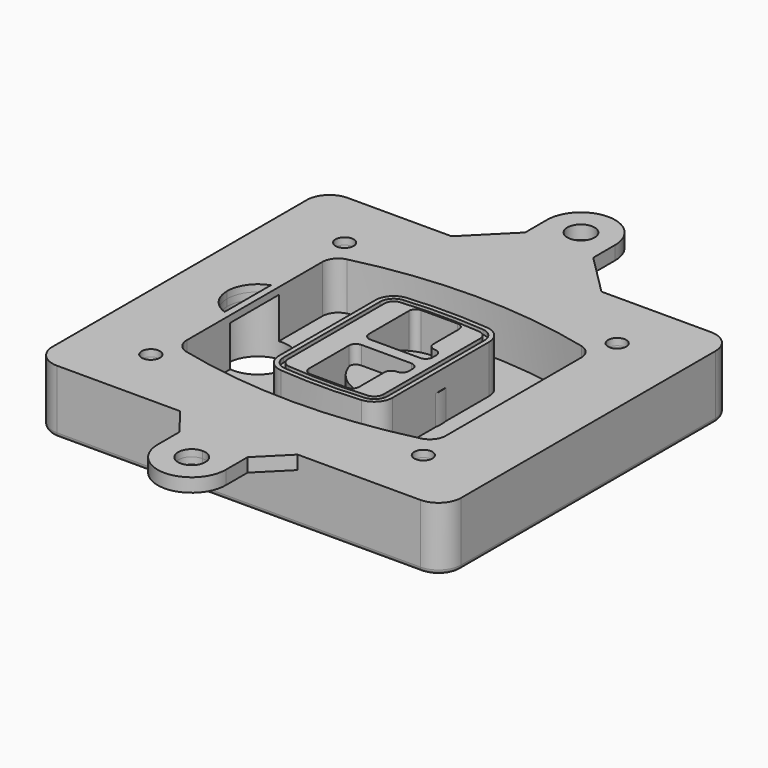
from build123d import *

# Parameters (mm, degrees)
F0_R      = 4
F1_DEPTH  = 25
F2_DEPTH  = 3
F3_DEPTH  = 18
F5_DEPTH  = 21
F6_DEPTH  = 2
F8_DEPTH  = 20
F9_DEPTH  = 16
F10_DEPTH = 25
F7_R      = 6
F7_R_2    = 4
F11_DEPTH = 6
F13_DEPTH = 9
F15_R     = 2
F16_R     = 4
F17_DEPTH = 3


# Not quite as in the source:
# - a feature of the source that left no trace in its solid (it failed there, or was rolled back) is left out
# - a feature names something its author has since deleted; it is built from what else it names


with BuildPart() as f1:
    # F0 (on Top) → F1 (new body)
    with BuildSketch(Plane.XY):
        with BuildLine():
            ThreePointArc((-90, -70), (-87.0710678119, -77.0710678119), (-80, -80))
            Line((-80, -80), (80, -80))
            ThreePointArc((80, -80), (87.0710678119, -77.0710678119), (90, -70))
            Line((90, -70), (90, 70))
            ThreePointArc((90, 70), (87.0710678119, 77.0710678119), (80, 80))
            Line((80, 80), (-80, 80))
            ThreePointArc((-80, 80), (-87.0710678119, 77.0710678119), (-90, 70))
            Line((-90, 70), (-90, -70))
        make_face()
        with Locations((-60, -53.3333333333)):
            Circle(F0_R, mode=Mode.SUBTRACT)
        with Locations((60, -53.3333333333)):
            Circle(F0_R, mode=Mode.SUBTRACT)
        with Locations((-60, 53.3333333333)):
            Circle(F0_R, mode=Mode.SUBTRACT)
        with BuildLine():
            ThreePointArc((-64, 37.2990447398), (-61.0143011354, 45.9411029726), (-53.3306899286, 50.8970778549))
            ThreePointArc((-53.3306899286, 50.8970778549), (0, 57.3333333333), (53.3306899286, 50.8970778549))
            ThreePointArc((53.3306899286, 50.8970778549), (61.0143011354, 45.9411029726), (64, 37.2990447398))
            Line((64, 37.2990447398), (64, -37.2990447398))
            ThreePointArc((64, -37.2990447398), (61.0143011354, -45.9411029726), (53.3306899286, -50.8970778549))
            ThreePointArc((53.3306899286, -50.8970778549), (0, -57.3333333333), (-53.3306899286, -50.8970778549))
            ThreePointArc((-53.3306899286, -50.8970778549), (-61.0143011354, -45.9411029726), (-64, -37.2990447398))
            Line((-64, -37.2990447398), (-64, 37.2990447398))
        make_face(mode=Mode.SUBTRACT)
        with Locations((60, 53.3333333333)):
            Circle(F0_R, mode=Mode.SUBTRACT)
        with BuildLine():
            ThreePointArc((53.3306899286, 50.8970778549), (0, 57.3333333333), (-53.3306899286, 50.8970778549))
            ThreePointArc((-53.3306899286, 50.8970778549), (-61.0143011354, 45.9411029726), (-64, 37.2990447398))
            Line((-64, 37.2990447398), (-64, -37.2990447398))
            ThreePointArc((-64, -37.2990447398), (-61.0143011354, -45.9411029726), (-53.3306899286, -50.8970778549))
            ThreePointArc((-53.3306899286, -50.8970778549), (0, -57.3333333333), (53.3306899286, -50.8970778549))
            ThreePointArc((53.3306899286, -50.8970778549), (61.0143011354, -45.9411029726), (64, -37.2990447398))
            Line((64, -37.2990447398), (64, 37.2990447398))
            ThreePointArc((64, 37.2990447398), (61.0143011354, 45.9411029726), (53.3306899286, 50.8970778549))
        make_face()
        with BuildLine():
            Line((-60, -37.2990447398), (-60, 37.2990447398))
            ThreePointArc((-60, 37.2990447398), (-57.8673579538, 43.4719434775), (-52.3790642347, 47.0119255363))
            ThreePointArc((-52.3790642347, 47.0119255363), (0, 53.3333333333), (52.3790642347, 47.0119255363))
            ThreePointArc((52.3790642347, 47.0119255363), (57.8673579538, 43.4719434775), (60, 37.2990447398))
            Line((60, 37.2990447398), (60, -37.2990447398))
            ThreePointArc((60, -37.2990447398), (57.8673579538, -43.4719434775), (52.3790642347, -47.0119255363))
            ThreePointArc((52.3790642347, -47.0119255363), (0, -53.3333333333), (-52.3790642347, -47.0119255363))
            ThreePointArc((-52.3790642347, -47.0119255363), (-57.8673579538, -43.4719434775), (-60, -37.2990447398))
        make_face(mode=Mode.SUBTRACT)
        with BuildLine():
            ThreePointArc((-52.3790642347, 47.0119255363), (-57.8673579538, 43.4719434775), (-60, 37.2990447398))
            Line((-60, 37.2990447398), (-60, -37.2990447398))
            ThreePointArc((-60, -37.2990447398), (-57.8673579538, -43.4719434775), (-52.3790642347, -47.0119255363))
            ThreePointArc((-52.3790642347, -47.0119255363), (0, -53.3333333333), (52.3790642347, -47.0119255363))
            ThreePointArc((52.3790642347, -47.0119255363), (57.8673579538, -43.4719434775), (60, -37.2990447398))
            Line((60, -37.2990447398), (60, 37.2990447398))
            ThreePointArc((60, 37.2990447398), (57.8673579538, 43.4719434775), (52.3790642347, 47.0119255363))
            ThreePointArc((52.3790642347, 47.0119255363), (0, 53.3333333333), (-52.3790642347, 47.0119255363))
        make_face()
        with BuildLine():
            ThreePointArc((51.6653449643, 44.0980612973), (55.5071505677, 41.6200738562), (57, 37.2990447398))
            Line((57, 37.2990447398), (57, -37.2990447398))
            ThreePointArc((57, -37.2990447398), (55.5071505677, -41.6200738562), (51.6653449643, -44.0980612973))
            ThreePointArc((51.6653449643, -44.0980612973), (0, -50.3333333333), (-51.6653449643, -44.0980612973))
            ThreePointArc((-51.6653449643, -44.0980612973), (-55.5071505677, -41.6200738562), (-57, -37.2990447398))
            Line((-57, -37.2990447398), (-57, 37.2990447398))
            ThreePointArc((-57, 37.2990447398), (-55.5071505677, 41.6200738562), (-51.6653449643, 44.0980612973))
            ThreePointArc((-51.6653449643, 44.0980612973), (0, 50.3333333333), (51.6653449643, 44.0980612973))
        make_face(mode=Mode.SUBTRACT)
        with BuildLine():
            Line((57, -37.2990447398), (57, 37.2990447398))
            ThreePointArc((57, 37.2990447398), (55.5071505677, 41.6200738562), (51.6653449643, 44.0980612973))
            ThreePointArc((51.6653449643, 44.0980612973), (0, 50.3333333333), (-51.6653449643, 44.0980612973))
            ThreePointArc((-51.6653449643, 44.0980612973), (-55.5071505677, 41.6200738562), (-57, 37.2990447398))
            Line((-57, 37.2990447398), (-57, -37.2990447398))
            ThreePointArc((-57, -37.2990447398), (-55.5071505677, -41.6200738562), (-51.6653449643, -44.0980612973))
            ThreePointArc((-51.6653449643, -44.0980612973), (0, -50.3333333333), (51.6653449643, -44.0980612973))
            ThreePointArc((51.6653449643, -44.0980612973), (55.5071505677, -41.6200738562), (57, -37.2990447398))
        make_face()
    extrude(amount=-F1_DEPTH)

    # F0 (on Top) → F2 (join)
    with BuildSketch(Plane.XY):
        with BuildLine():
            ThreePointArc((-52.3790642347, 47.0119255363), (-57.8673579538, 43.4719434775), (-60, 37.2990447398))
            Line((-60, 37.2990447398), (-60, -37.2990447398))
            ThreePointArc((-60, -37.2990447398), (-57.8673579538, -43.4719434775), (-52.3790642347, -47.0119255363))
            ThreePointArc((-52.3790642347, -47.0119255363), (0, -53.3333333333), (52.3790642347, -47.0119255363))
            ThreePointArc((52.3790642347, -47.0119255363), (57.8673579538, -43.4719434775), (60, -37.2990447398))
            Line((60, -37.2990447398), (60, 37.2990447398))
            ThreePointArc((60, 37.2990447398), (57.8673579538, 43.4719434775), (52.3790642347, 47.0119255363))
            ThreePointArc((52.3790642347, 47.0119255363), (0, 53.3333333333), (-52.3790642347, 47.0119255363))
        make_face()
        with BuildLine():
            ThreePointArc((51.6653449643, 44.0980612973), (55.5071505677, 41.6200738562), (57, 37.2990447398))
            Line((57, 37.2990447398), (57, -37.2990447398))
            ThreePointArc((57, -37.2990447398), (55.5071505677, -41.6200738562), (51.6653449643, -44.0980612973))
            ThreePointArc((51.6653449643, -44.0980612973), (0, -50.3333333333), (-51.6653449643, -44.0980612973))
            ThreePointArc((-51.6653449643, -44.0980612973), (-55.5071505677, -41.6200738562), (-57, -37.2990447398))
            Line((-57, -37.2990447398), (-57, 37.2990447398))
            ThreePointArc((-57, 37.2990447398), (-55.5071505677, 41.6200738562), (-51.6653449643, 44.0980612973))
            ThreePointArc((-51.6653449643, 44.0980612973), (0, 50.3333333333), (51.6653449643, 44.0980612973))
        make_face(mode=Mode.SUBTRACT)
    extrude(amount=F2_DEPTH)

    # F0 (on Top) → F3 (cut)
    with BuildSketch(Plane.XY):
        with BuildLine():
            Line((57, -37.2990447398), (57, 37.2990447398))
            ThreePointArc((57, 37.2990447398), (55.5071505677, 41.6200738562), (51.6653449643, 44.0980612973))
            ThreePointArc((51.6653449643, 44.0980612973), (0, 50.3333333333), (-51.6653449643, 44.0980612973))
            ThreePointArc((-51.6653449643, 44.0980612973), (-55.5071505677, 41.6200738562), (-57, 37.2990447398))
            Line((-57, 37.2990447398), (-57, -37.2990447398))
            ThreePointArc((-57, -37.2990447398), (-55.5071505677, -41.6200738562), (-51.6653449643, -44.0980612973))
            ThreePointArc((-51.6653449643, -44.0980612973), (0, -50.3333333333), (51.6653449643, -44.0980612973))
            ThreePointArc((51.6653449643, -44.0980612973), (55.5071505677, -41.6200738562), (57, -37.2990447398))
        make_face()
    extrude(amount=-F3_DEPTH, mode=Mode.SUBTRACT)

    # F4 (on face) → F5 (join, through all)
    with BuildSketch(Plane.XY.offset(3)):
        with BuildLine():
            ThreePointArc((-25, -26.587695628), (-22.8992979869, -31.9912392117), (-17.7004291845, -34.5569740744))
            ThreePointArc((-17.7004291845, -34.5569740744), (0, -35.3333333333), (17.7004291845, -34.5569740744))
            ThreePointArc((17.7004291845, -34.5569740744), (22.8992979869, -31.9912392117), (25, -26.587695628))
            Line((25, -26.587695628), (25, 26.587695628))
            ThreePointArc((25, 26.587695628), (22.8992979869, 31.9912392117), (17.7004291845, 34.5569740744))
            ThreePointArc((17.7004291845, 34.5569740744), (0, 35.3333333333), (-17.7004291845, 34.5569740744))
            ThreePointArc((-17.7004291845, 34.5569740744), (-22.8992979869, 31.9912392117), (-25, 26.587695628))
            Line((-25, 26.587695628), (-25, -26.587695628))
        make_face()
        with BuildLine():
            ThreePointArc((17.5253218884, 32.5646544628), (21.4244734902, 30.6403533158), (23, 26.587695628))
            Line((23, 26.587695628), (23, -26.587695628))
            ThreePointArc((23, -26.587695628), (21.4244734902, -30.6403533158), (17.5253218884, -32.5646544628))
            ThreePointArc((17.5253218884, -32.5646544628), (0, -33.3333333333), (-17.5253218884, -32.5646544628))
            ThreePointArc((-17.5253218884, -32.5646544628), (-21.4244734902, -30.6403533158), (-23, -26.587695628))
            Line((-23, -26.587695628), (-23, 26.587695628))
            ThreePointArc((-23, 26.587695628), (-21.4244734902, 30.6403533158), (-17.5253218884, 32.5646544628))
            ThreePointArc((-17.5253218884, 32.5646544628), (0, 33.3333333333), (17.5253218884, 32.5646544628))
        make_face(mode=Mode.SUBTRACT)
        with BuildLine():
            Line((23, -26.587695628), (23, 26.587695628))
            ThreePointArc((23, 26.587695628), (21.4244734902, 30.6403533158), (17.5253218884, 32.5646544628))
            ThreePointArc((17.5253218884, 32.5646544628), (0, 33.3333333333), (-17.5253218884, 32.5646544628))
            ThreePointArc((-17.5253218884, 32.5646544628), (-21.4244734902, 30.6403533158), (-23, 26.587695628))
            Line((-23, 26.587695628), (-23, -26.587695628))
            ThreePointArc((-23, -26.587695628), (-21.4244734902, -30.6403533158), (-17.5253218884, -32.5646544628))
            ThreePointArc((-17.5253218884, -32.5646544628), (0, -33.3333333333), (17.5253218884, -32.5646544628))
            ThreePointArc((17.5253218884, -32.5646544628), (21.4244734902, -30.6403533158), (23, -26.587695628))
        make_face()
        with BuildLine():
            ThreePointArc((17.3502145923, 30.5723348512), (19.9496489934, 29.2894674198), (21, 26.587695628))
            Line((21, 26.587695628), (21, -26.587695628))
            ThreePointArc((21, -26.587695628), (19.9496489934, -29.2894674198), (17.3502145923, -30.5723348512))
            ThreePointArc((17.3502145923, -30.5723348512), (0, -31.3333333333), (-17.3502145923, -30.5723348512))
            ThreePointArc((-17.3502145923, -30.5723348512), (-19.9496489934, -29.2894674198), (-21, -26.587695628))
            Line((-21, -26.587695628), (-21, 26.587695628))
            ThreePointArc((-21, 26.587695628), (-19.9496489934, 29.2894674198), (-17.3502145923, 30.5723348512))
            ThreePointArc((-17.3502145923, 30.5723348512), (0, 31.3333333333), (17.3502145923, 30.5723348512))
        make_face(mode=Mode.SUBTRACT)
        with BuildLine():
            Line((21, -26.587695628), (21, 26.587695628))
            ThreePointArc((21, 26.587695628), (19.9496489934, 29.2894674198), (17.3502145923, 30.5723348512))
            ThreePointArc((17.3502145923, 30.5723348512), (0, 31.3333333333), (-17.3502145923, 30.5723348512))
            ThreePointArc((-17.3502145923, 30.5723348512), (-19.9496489934, 29.2894674198), (-21, 26.587695628))
            Line((-21, 26.587695628), (-21, -26.587695628))
            ThreePointArc((-21, -26.587695628), (-19.9496489934, -29.2894674198), (-17.3502145923, -30.5723348512))
            ThreePointArc((-17.3502145923, -30.5723348512), (0, -31.3333333333), (17.3502145923, -30.5723348512))
            ThreePointArc((17.3502145923, -30.5723348512), (19.9496489934, -29.2894674198), (21, -26.587695628))
        make_face()
        with BuildLine():
            Line((-8, -2.5), (14, -2.5))
            ThreePointArc((14, -2.5), (16.1213203436, -3.3786796564), (17, -5.5))
            Line((17, -5.5), (17, -7.5))
            ThreePointArc((17, -7.5), (16.1213203436, -9.6213203436), (14, -10.5))
            ThreePointArc((14, -10.5), (11.8786796564, -11.3786796564), (11, -13.5))
            Line((11, -13.5), (11, -27.5))
            ThreePointArc((11, -27.5), (10.1213203436, -29.6213203436), (8, -30.5))
            Line((8, -30.5), (-8, -30.5))
            ThreePointArc((-8, -30.5), (-10.1213203436, -29.6213203436), (-11, -27.5))
            Line((-11, -27.5), (-11, -5.5))
            ThreePointArc((-11, -5.5), (-10.1213203436, -3.3786796564), (-8, -2.5))
        make_face(mode=Mode.SUBTRACT)
        with BuildLine():
            ThreePointArc((-8, 2.5), (-10.1213203436, 3.3786796564), (-11, 5.5))
            Line((-11, 5.5), (-11, 27.5))
            ThreePointArc((-11, 27.5), (-10.1213203436, 29.6213203436), (-8, 30.5))
            Line((-8, 30.5), (8, 30.5))
            ThreePointArc((8, 30.5), (10.1213203436, 29.6213203436), (11, 27.5))
            Line((11, 27.5), (11, 13.5))
            ThreePointArc((11, 13.5), (11.8786796564, 11.3786796564), (14, 10.5))
            ThreePointArc((14, 10.5), (16.1213203436, 9.6213203436), (17, 7.5))
            Line((17, 7.5), (17, 5.5))
            ThreePointArc((17, 5.5), (16.1213203436, 3.3786796564), (14, 2.5))
            Line((14, 2.5), (-8, 2.5))
        make_face(mode=Mode.SUBTRACT)
    extrude(amount=-F5_DEPTH)

    # F4 (on face) → F6 (cut)
    with BuildSketch(Plane.XY.offset(3)):
        with BuildLine():
            Line((23, -26.587695628), (23, 26.587695628))
            ThreePointArc((23, 26.587695628), (21.4244734902, 30.6403533158), (17.5253218884, 32.5646544628))
            ThreePointArc((17.5253218884, 32.5646544628), (0, 33.3333333333), (-17.5253218884, 32.5646544628))
            ThreePointArc((-17.5253218884, 32.5646544628), (-21.4244734902, 30.6403533158), (-23, 26.587695628))
            Line((-23, 26.587695628), (-23, -26.587695628))
            ThreePointArc((-23, -26.587695628), (-21.4244734902, -30.6403533158), (-17.5253218884, -32.5646544628))
            ThreePointArc((-17.5253218884, -32.5646544628), (0, -33.3333333333), (17.5253218884, -32.5646544628))
            ThreePointArc((17.5253218884, -32.5646544628), (21.4244734902, -30.6403533158), (23, -26.587695628))
        make_face()
        with BuildLine():
            ThreePointArc((17.3502145923, 30.5723348512), (19.9496489934, 29.2894674198), (21, 26.587695628))
            Line((21, 26.587695628), (21, -26.587695628))
            ThreePointArc((21, -26.587695628), (19.9496489934, -29.2894674198), (17.3502145923, -30.5723348512))
            ThreePointArc((17.3502145923, -30.5723348512), (0, -31.3333333333), (-17.3502145923, -30.5723348512))
            ThreePointArc((-17.3502145923, -30.5723348512), (-19.9496489934, -29.2894674198), (-21, -26.587695628))
            Line((-21, -26.587695628), (-21, 26.587695628))
            ThreePointArc((-21, 26.587695628), (-19.9496489934, 29.2894674198), (-17.3502145923, 30.5723348512))
            ThreePointArc((-17.3502145923, 30.5723348512), (0, 31.3333333333), (17.3502145923, 30.5723348512))
        make_face(mode=Mode.SUBTRACT)
    extrude(amount=-F6_DEPTH, mode=Mode.SUBTRACT)

    # F7 (on face) → F8 (join)
    with BuildSketch(Plane(origin=(0, 0, -25), x_dir=(1, 0, 0), z_dir=(0, 0, -1))):
        with BuildLine():
            ThreePointArc((-6.71157564, 0), (6.7567035675, 13.4682792075), (20.224982775, 0))
            Line((20.224982775, 0), (25.224982775, 0))
            ThreePointArc((25.224982775, 0), (6.7567035675, 18.4682792075), (-11.71157564, 0))
            Line((-11.71157564, 0), (-6.71157564, 0))
        make_face()
        with BuildLine():
            Line((-6.71157564, 0), (20.224982775, 0))
            ThreePointArc((20.224982775, 0), (6.7567035675, 13.4682792075), (-6.71157564, 0))
        make_face()
        with BuildLine():
            ThreePointArc((-6.71157564, 0), (6.7567035675, -13.4682792075), (20.224982775, 0))
            Line((20.224982775, 0), (-6.71157564, 0))
        make_face()
        with BuildLine():
            Line((25.224982775, 0), (20.224982775, 0))
            ThreePointArc((20.224982775, 0), (6.7567035675, -13.4682792075), (-6.71157564, 0))
            Line((-6.71157564, 0), (-11.71157564, 0))
            ThreePointArc((-11.71157564, 0), (6.7567035675, -18.4682792075), (25.224982775, 0))
        make_face()
    extrude(amount=-F8_DEPTH)

    # F7 (on face) → F9 (cut)
    with BuildSketch(Plane(origin=(0, 0, -25), x_dir=(1, 0, 0), z_dir=(0, 0, -1))):
        with BuildLine():
            Line((-6.71157564, 0), (20.224982775, 0))
            ThreePointArc((20.224982775, 0), (6.7567035675, 13.4682792075), (-6.71157564, 0))
        make_face()
        with BuildLine():
            ThreePointArc((-6.71157564, 0), (6.7567035675, -13.4682792075), (20.224982775, 0))
            Line((20.224982775, 0), (-6.71157564, 0))
        make_face()
    extrude(amount=-F9_DEPTH, mode=Mode.SUBTRACT)

    # F7 (on face) → F10 (cut)
    with BuildSketch(Plane(origin=(0, 0, -25), x_dir=(1, 0, 0), z_dir=(0, 0, -1))):
        with BuildLine():
            Line((-69.0318229325, 0), (-42.0952645175, 0))
            ThreePointArc((-42.0952645175, 0), (-55.563543725, 13.4682792075), (-69.0318229325, 0))
        make_face()
        with BuildLine():
            ThreePointArc((-69.0318229325, 0), (-55.563543725, -13.4682792075), (-42.0952645175, 0))
            Line((-42.0952645175, 0), (-69.0318229325, 0))
        make_face()
    extrude(amount=-F10_DEPTH, mode=Mode.SUBTRACT)

    # F7 (on face) → F11 (cut)
    with BuildSketch(Plane(origin=(0, 0, -25), x_dir=(1, 0, 0), z_dir=(0, 0, -1))):
        with Locations((60, -53.3333333333)):
            Circle(F7_R)
        with Locations((60, -53.3333333333)):
            Circle(F7_R_2, mode=Mode.SUBTRACT)
        with Locations((-60, -53.3333333333)):
            Circle(F7_R)
        with Locations((-60, -53.3333333333)):
            Circle(F7_R_2, mode=Mode.SUBTRACT)
        with Locations((-60, 53.3333333333)):
            Circle(F7_R)
        with Locations((-60, 53.3333333333)):
            Circle(F7_R_2, mode=Mode.SUBTRACT)
        with Locations((60, 53.3333333333)):
            Circle(F7_R)
        with Locations((60, 53.3333333333)):
            Circle(F7_R_2, mode=Mode.SUBTRACT)
    extrude(amount=-F11_DEPTH, mode=Mode.SUBTRACT)

    # F12 (on face) → F13 (cut, through all)
    with BuildSketch(Plane(origin=(0, 0, -9), x_dir=(1, 0, 0), z_dir=(0, 0, -1))):
        with BuildLine():
            ThreePointArc((20.224982775, 0), (20.1663399806, 1.2554664788), (19.9909222755, 2.5))
            Line((19.9909222755, 2.5), (14, 2.5))
            ThreePointArc((14, 2.5), (16.1213203436, 3.3786796564), (17, 5.5))
            Line((17, 5.5), (17, 7.5))
            ThreePointArc((17, 7.5), (16.1213203436, 9.6213203436), (14, 10.5))
            ThreePointArc((14, 10.5), (12.1627255951, 11.1284134507), (11.0951631559, 12.750384826))
            ThreePointArc((11.0951631559, 12.750384826), (11.0476113807, 12.7664660322), (11, 12.7823698976))
            Line((11, 12.7823698976), (11, -12.7823698976))
            ThreePointArc((11, -12.7823698976), (11.0476113807, -12.7664660322), (11.0951631559, -12.750384826))
            ThreePointArc((11.0951631559, -12.750384826), (12.1627255951, -11.1284134507), (14, -10.5))
            ThreePointArc((14, -10.5), (16.1213203436, -9.6213203436), (17, -7.5))
            Line((17, -7.5), (17, -5.5))
            ThreePointArc((17, -5.5), (16.1213203436, -3.3786796564), (14, -2.5))
            Line((14, -2.5), (19.9909222755, -2.5))
            ThreePointArc((19.9909222755, -2.5), (20.1663399806, -1.2554664788), (20.224982775, 0))
        make_face()
    extrude(amount=F13_DEPTH, mode=Mode.SUBTRACT)

    # F15
    f15_edges = [f1.edges().sort_by_distance(p)[0] for p in [
        (0, -80, -25),
        (-87.071068, -77.071068, -25),
        (-90, 0, -25),
        (-87.071068, 77.071068, -25),
        (87.071068, -77.071068, -25),
        (0, 80, -25),
        (90, 0, -25),
        (87.071068, 77.071068, -25),
    ]]
    fillet(f15_edges, radius=F15_R)

    # F16 (on face) → F17 (join, symmetric)
    with BuildSketch(Plane.XY):
        with BuildLine():
            Line((-16.262158438, 98), (-34.262158438, 80))
            Line((-34.262158438, 80), (-1.2684588879, 80))
            Line((-1.2684588879, 80), (31.7315411121, 80))
            Line((31.7315411121, 80), (13.7315411121, 98))
            Line((13.7315411121, 98), (13.7315411121, 110))
            ThreePointArc((13.7315411121, 110), (-1.4858373008, 124.9984248048), (-16.262158438, 109.5652888294))
            Line((-16.262158438, 109.5652888294), (-16.262158438, 98))
        make_face()
        with BuildLine():
            ThreePointArc((4.7315411121, 110), (2.9741817992, 105.7573593129), (-1.2684588879, 104))
            ThreePointArc((-1.2684588879, 104), (-5.5110995751, 114.2426406871), (4.7315411121, 110))
        make_face(mode=Mode.SUBTRACT)
        with BuildLine():
            Line((-1.2684588879, 80), (-34.262158438, 80))
            Line((-34.262158438, 80), (-80, 80))
            ThreePointArc((-80, 80), (-87.0710678119, 77.0710678119), (-90, 70))
            Line((-90, 70), (-90, -70))
            ThreePointArc((-90, -70), (-87.0710678119, -77.0710678119), (-80, -80))
            Line((-80, -80), (-25.7836213731, -80))
            Line((-25.7836213731, -80), (-1.2684588879, -80))
            Line((-1.2684588879, -80), (25.9815411121, -80))
            Line((25.9815411121, -80), (80, -80))
            ThreePointArc((80, -80), (87.0710678119, -77.0710678119), (90, -70))
            Line((90, -70), (90, 70))
            ThreePointArc((90, 70), (87.0710678119, 77.0710678119), (80, 80))
            Line((80, 80), (31.7315411121, 80))
            Line((31.7315411121, 80), (-1.2684588879, 80))
        make_face()
        with Locations((-60, -53.3333333333)):
            Circle(F16_R, mode=Mode.SUBTRACT)
        with BuildLine():
            Line((-60, 12.7166190685), (-60, 37.2990447398))
            ThreePointArc((-60, 37.2990447398), (-57.8673579538, 43.4719434775), (-52.3790642347, 47.0119255363))
            ThreePointArc((-52.3790642347, 47.0119255363), (0, 53.3333333333), (52.3790642347, 47.0119255363))
            ThreePointArc((52.3790642347, 47.0119255363), (57.8673579538, 43.4719434775), (60, 37.2990447398))
            Line((60, 37.2990447398), (60, -37.2990447398))
            ThreePointArc((60, -37.2990447398), (57.8673579538, -43.4719434775), (52.3790642347, -47.0119255363))
            ThreePointArc((52.3790642347, -47.0119255363), (0, -53.3333333333), (-52.3790642347, -47.0119255363))
            ThreePointArc((-52.3790642347, -47.0119255363), (-57.8673579538, -43.4719434775), (-60, -37.2990447398))
            Line((-60, -37.2990447398), (-60, -12.7166190685))
            ThreePointArc((-60, -12.7166190685), (-66.5441169481, -7.798817635), (-69.0318229325, 0))
            ThreePointArc((-69.0318229325, 0), (-66.5441169481, 7.798817635), (-60, 12.7166190685))
        make_face(mode=Mode.SUBTRACT)
        with Locations((60, -53.3333333333)):
            Circle(F16_R, mode=Mode.SUBTRACT)
        with Locations((-60, 53.3333333333)):
            Circle(F16_R, mode=Mode.SUBTRACT)
        with Locations((60, 53.3333333333)):
            Circle(F16_R, mode=Mode.SUBTRACT)
        with BuildLine():
            Line((-1.2684588879, -80), (-25.7836213731, -80))
            Line((-25.7836213731, -80), (-16.262158438, -92.25))
            Line((-16.262158438, -92.25), (-16.262158438, -103.8152888294))
            ThreePointArc((-16.262158438, -103.8152888294), (-1.4858373008, -119.2484248048), (13.7315411121, -104.25))
            Line((13.7315411121, -104.25), (13.7315411121, -92.25))
            Line((13.7315411121, -92.25), (25.9815411121, -80))
            Line((25.9815411121, -80), (-1.2684588879, -80))
        make_face()
        with BuildLine():
            ThreePointArc((4.7315411121, -104.25), (-5.5110995751, -108.4926406871), (-1.2684588879, -98.25))
            ThreePointArc((-1.2684588879, -98.25), (2.9741817992, -100.0073593129), (4.7315411121, -104.25))
        make_face(mode=Mode.SUBTRACT)
    extrude(amount=F17_DEPTH, both=True)


solid = f1.part
